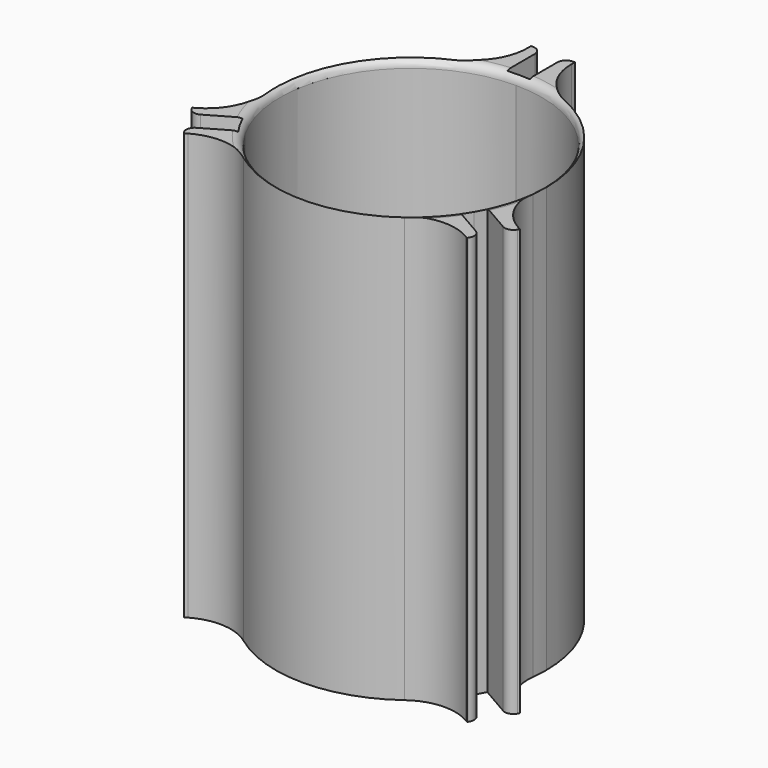
from build123d import *

# Parameters (mm, degrees)
F1_DEPTH = 50.8
F2_R     = 6.35
F3_R     = 1.016


# Not quite as in the source:
# - a fillet or chamfer that OpenCascade refuses, or shapes differently, is made with other operations: its cross-section is extruded or revolved along the edge and cut away or added


with BuildPart() as f1:
    # F0 (on Top) → F1 (new body)
    with BuildSketch(Plane.XY):
        with BuildLine():
            ThreePointArc((-2.6150272293, 15.9155984364), (-1.9815871124, 16.0068095983), (-1.3450272293, 16.07282))
            Line((-1.3450272293, 16.07282), (-1.3450272293, 21.15282))
            Line((-1.3450272293, 21.15282), (-2.6150272293, 21.15282))
            Line((-2.6150272293, 21.15282), (-2.6150272293, 15.9155984364))
        make_face()
        with BuildLine():
            Line((1.3450272293, 21.15282), (1.3450272293, 16.07282))
            ThreePointArc((1.3450272293, 16.07282), (1.9815871124, 16.0068095983), (2.6150272293, 15.9155984364))
            Line((2.6150272293, 15.9155984364), (2.6150272293, 21.15282))
            Line((2.6150272293, 21.15282), (1.3450272293, 21.15282))
        make_face()
        with BuildLine():
            ThreePointArc((0, 15.621), (11.0457150289, 11.0457150289), (15.621, 0))
            ThreePointArc((15.621, 0), (15.0887273325, -4.0430123035), (13.5281828325, -7.8105))
            Line((13.5281828325, -7.8105), (13.9681237376, -8.0645))
            ThreePointArc((13.9681237376, -8.0645), (14.2925051104, -7.4745527405), (14.5919840451, -6.8715822506))
            ThreePointArc((14.5919840451, -6.8715822506), (14.8530973018, -6.28730002), (15.090826177, -5.693119206))
            ThreePointArc((15.090826177, -5.693119206), (15.867333998, -2.8935018222), (16.129, 0))
            ThreePointArc((16.129, 0), (12.2947634215, 10.439513083), (2.6150272293, 15.9155984364))
            ThreePointArc((2.6150272293, 15.9155984364), (1.9815871124, 16.0068095983), (1.3450272293, 16.07282))
            ThreePointArc((1.3450272293, 16.07282), (0.6731, 16.1149488795), (0, 16.129))
            Line((0, 16.129), (0, 15.621))
        make_face()
        with BuildLine():
            ThreePointArc((15.090826177, -5.693119206), (14.8530973018, -6.28730002), (14.5919840451, -6.8715822506))
            Line((14.5919840451, -6.8715822506), (18.9913930963, -9.4115822506))
            Line((18.9913930963, -9.4115822506), (19.6263930963, -8.3117299878))
            Line((19.6263930963, -8.3117299878), (15.090826177, -5.693119206))
        make_face()
        with BuildLine():
            Line((17.646365867, -11.7412377494), (13.2469568158, -9.2012377494))
            ThreePointArc((13.2469568158, -9.2012377494), (12.8744329677, -9.7156377434), (12.4819459699, -10.2149726287))
            Line((12.4819459699, -10.2149726287), (16.8813550211, -12.7549726287))
            Line((16.8813550211, -12.7549726287), (17.646365867, -11.7412377494))
        make_face()
        with BuildLine():
            Line((13.9681237376, -8.0645), (13.5281828325, -7.8105))
            ThreePointArc((13.5281828325, -7.8105), (0, -15.621), (-13.5281828325, -7.8105))
            Line((-13.5281828325, -7.8105), (-13.9681237376, -8.0645))
            ThreePointArc((-13.9681237376, -8.0645), (-13.6194051104, -8.6403961391), (-13.2469568158, -9.2012377494))
            ThreePointArc((-13.2469568158, -9.2012377494), (-12.8744329677, -9.7156377434), (-12.4819459699, -10.2149726287))
            ThreePointArc((-12.4819459699, -10.2149726287), (0, -16.129), (12.4819459699, -10.2149726287))
            ThreePointArc((12.4819459699, -10.2149726287), (12.8744329677, -9.7156377434), (13.2469568158, -9.2012377494))
            ThreePointArc((13.2469568158, -9.2012377494), (13.6194051104, -8.6403961391), (13.9681237376, -8.0645))
        make_face()
        with BuildLine():
            ThreePointArc((-12.4819459699, -10.2149726287), (-12.8744329677, -9.7156377434), (-13.2469568158, -9.2012377494))
            Line((-13.2469568158, -9.2012377494), (-17.646365867, -11.7412377494))
            Line((-17.646365867, -11.7412377494), (-16.8813550211, -12.7549726287))
            Line((-16.8813550211, -12.7549726287), (-12.4819459699, -10.2149726287))
        make_face()
        with BuildLine():
            ThreePointArc((-13.5281828325, -7.8105), (-13.5281828325, 7.8105), (0, 15.621))
            Line((0, 15.621), (0, 16.129))
            ThreePointArc((0, 16.129), (-0.6731, 16.1149488795), (-1.3450272293, 16.07282))
            ThreePointArc((-1.3450272293, 16.07282), (-1.9815871124, 16.0068095983), (-2.6150272293, 15.9155984364))
            ThreePointArc((-2.6150272293, 15.9155984364), (-13.970548685, 8.0602984088), (-15.0873987804, -5.7021959842))
            ThreePointArc((-15.0873987804, -5.7021959842), (-14.8512055836, -6.2917671377), (-14.5919840451, -6.8715822506))
            ThreePointArc((-14.5919840451, -6.8715822506), (-14.2925051104, -7.4745527405), (-13.9681237376, -8.0645))
            Line((-13.9681237376, -8.0645), (-13.5281828325, -7.8105))
        make_face()
        with BuildLine():
            Line((-18.9913930963, -9.4115822506), (-14.5919840451, -6.8715822506))
            ThreePointArc((-14.5919840451, -6.8715822506), (-14.8512055836, -6.2917671377), (-15.0873987804, -5.7021959842))
            Line((-15.0873987804, -5.7021959842), (-19.4868078316, -8.2421959842))
            Line((-19.4868078316, -8.2421959842), (-18.9913930963, -9.4115822506))
        make_face()
    extrude(amount=F1_DEPTH)

    # F2
    f2_edges = [f1.edges().sort_by_distance(p)[0] for p in [
        (2.615027, 15.915598, 25.4),
        (15.090826, -5.693119, 25.4),
        (12.481946, -10.214973, 25.4),
        (-12.481946, -10.214973, 25.4),
        (-15.087399, -5.702196, 25.4),
        (-2.615027, 15.915598, 25.4),
    ]]
    fillet(f2_edges, radius=F2_R)

    # F3
    f3_edges = [f1.edges().sort_by_distance(p)[0] for p in [
        (1.345027, 21.15282, 25.4),
        (-1.345027, 21.15282, 25.4),
        (-18.991393, -9.411582, 25.4),
        (-17.646366, -11.741238, 25.4),
        (17.646366, -11.741238, 25.4),
        (18.991393, -9.411582, 25.4),
    ]]
    fillet(f3_edges, radius=F3_R)

    # F4: fillet of radius 1.016 on 1 edges, made by hand

    # F4_s1 → F4_t2 (revolve, cut)
    with BuildSketch(Plane.YZ):
        with BuildLine():
            ThreePointArc((15.621, 49.784), (15.9185795103, 50.5024204897), (16.637, 50.8))
            Line((16.637, 50.8), (15.621, 50.8))
            Line((15.621, 50.8), (15.621, 49.784))
        make_face()
    revolve(axis=Axis((0, 0, 50.8), (0, 0, -1)), mode=Mode.SUBTRACT)


solid = f1.part
